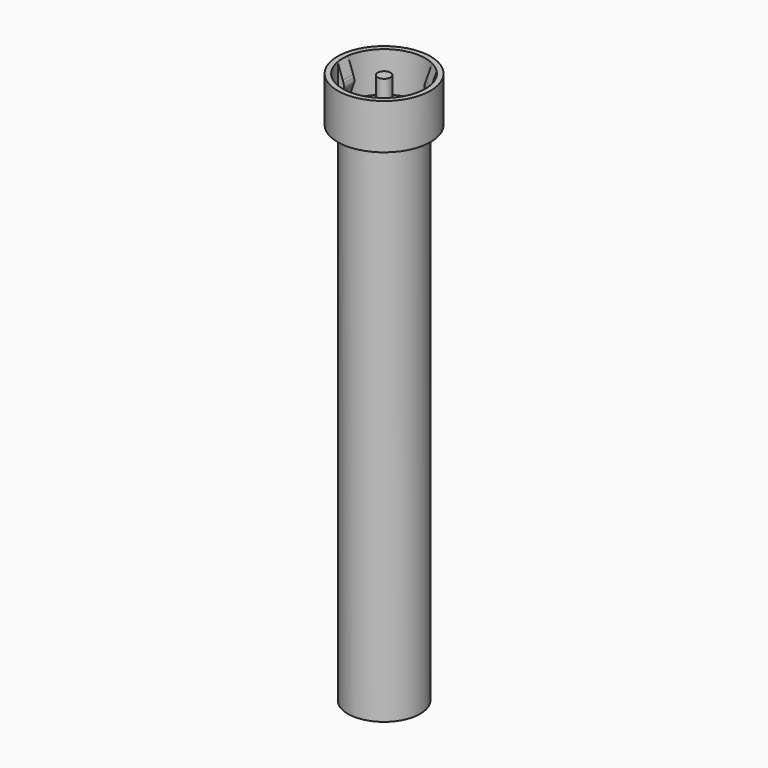
from build123d import *

# Parameters (mm, degrees)
F0_R             = 5.6
F1_DEPTH         = 78
F2_T             = -0.8
F3_R             = 1
F4_DEPTH         = 1
F6_R             = 7.2
F7_DEPTH         = 7
F8_T             = -0.8
F10_DEPTH        = 1
F10_DEPTH_BACK   = 1
F10_COPIES_COUNT = 3
F10_COPIES_ANGLE = 249
F11_R            = 1
F12_DEPTH        = 6


# Not quite as in the source:
# - a pattern or mirror of a feature is missing from the dataset's text; its kind, count and spacing are read off the source's solid


with BuildPart() as f1:
    # F0 (on Top) → F1 (new body)
    with BuildSketch(Plane.XY):
        Circle(F0_R)
    extrude(amount=F1_DEPTH)

    # F2
    f2_openings = [f1.faces().sort_by_distance(p)[0] for p in [
        (0, 0, 78),
    ]]
    offset(amount=F2_T, openings=f2_openings)

    # F3 (on face) → F4 (join)
    with BuildSketch(Plane.XY.offset(0.8)):
        Circle(F3_R)
    extrude(amount=F4_DEPTH)


with BuildPart() as f7:
    # F6 (on offset) → F7 (new body)
    with BuildSketch(Plane.XY.offset(78.5)):
        Circle(F6_R)
    extrude(amount=F7_DEPTH)

    # F8
    f8_openings = [f7.faces().sort_by_distance(p)[0] for p in [
        (0, 0, 85.5),
    ]]
    offset(amount=F8_T, openings=f8_openings)

    # F9 (on Front) → F10 (join, two sides)
    with BuildSketch(Plane.XZ) as f10_sk:
        Polygon((-6.4, 85.5), (-6.4, 79.3), (-5.6, 81.6190695472), (-5.6, 83.1809304528), align=None)
        with BuildLine():
            Line((-5.6, 83.1809304528), (-5.6, 81.6190695472))
            Line((-5.6, 81.6190695472), (-5.4656007986, 82.0086709162))
            ThreePointArc((-5.4656007986, 82.0086709162), (-5.4, 82.4), (-5.4656007986, 82.7913290838))
            Line((-5.4656007986, 82.7913290838), (-5.6, 83.1809304528))
        make_face()
    f10 = extrude(amount=F10_DEPTH) + extrude(f10_sk.sketch, amount=-F10_DEPTH_BACK)

    # F10_copies: F10 ×3 about axis
    f10_copies_axis = Axis((0, 0, 0), (0, 0, -1))
    for i in range(1, F10_COPIES_COUNT):
        add(f10.rotate(f10_copies_axis, i * F10_COPIES_ANGLE / (F10_COPIES_COUNT - 1)))

    # F11 (on face) → F12 (join)
    with BuildSketch(Plane.XY.offset(79.3)):
        Circle(F11_R)
    extrude(amount=F12_DEPTH)


solid = Compound([f1.part, f7.part])
